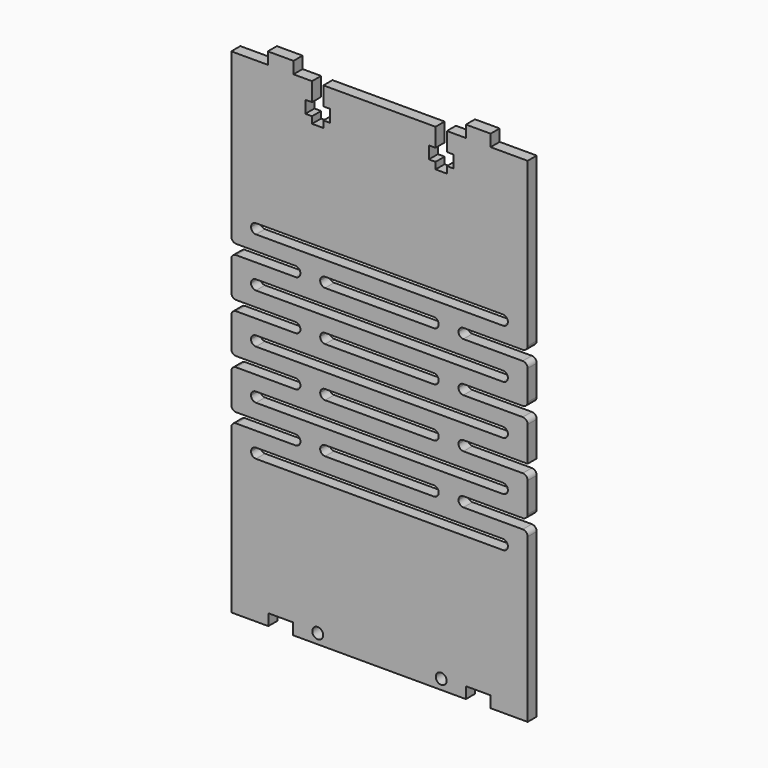
from build123d import *

# Parameters (mm, degrees)
F0_R     = 1.397
F1_DEPTH = 2.921
F2_R     = 1.26999


# Not quite as in the source:
# - a fillet or chamfer is up to 0.001 mm smaller than in the source, because OpenCascade refuses the exact size


with BuildPart() as f1:
    # F0 (on Front) → F1 (new body)
    with BuildSketch(Plane.XZ):
        Polygon((38.1, 68.58), (38.1, 64.77), (71.12, 64.77), (71.12, 63.5), (76.2, 63.5), (76.2, 68.58), (58.42, 68.58), (58.42, 71.12), (76.2, 71.12), (76.2, 81.28), (58.42, 81.28), (58.42, 83.82), (76.2, 83.82), (76.2, 127), (66.675, 127), (66.675, 123.952), (60.325, 123.952), (60.325, 127), (55.4355, 127), (55.4355, 122.2375), (57.15, 122.2375), (57.15, 119.0625), (55.4355, 119.0625), (55.4355, 117.348), (53.975, 117.348), (52.5145, 117.348), (52.5145, 119.0625), (50.8, 119.0625), (50.8, 122.2375), (52.5145, 122.2375), (52.5145, 127), (38.1, 127), (38.1, 90.17), (71.12, 90.17), (71.12, 87.63), (38.1, 87.63), (38.1, 83.82), (53.34, 83.82), (53.34, 81.28), (38.1, 81.28), (38.1, 77.47), (71.12, 77.47), (71.12, 74.93), (38.1, 74.93), (38.1, 71.12), (53.34, 71.12), (53.34, 68.58), align=None)
        Polygon((0, 68.58), (0, 63.5), (5.08, 63.5), (5.08, 64.77), (38.1, 64.77), (38.1, 68.58), (22.86, 68.58), (22.86, 71.12), (38.1, 71.12), (38.1, 74.93), (5.08, 74.93), (5.08, 77.47), (38.1, 77.47), (38.1, 81.28), (22.86, 81.28), (22.86, 83.82), (38.1, 83.82), (38.1, 87.63), (5.08, 87.63), (5.08, 90.17), (38.1, 90.17), (38.1, 127), (23.6855, 127), (23.6855, 122.2375), (25.4, 122.2375), (25.4, 119.0625), (23.6855, 119.0625), (23.6855, 117.348), (22.225, 117.348), (20.7645, 117.348), (20.7645, 119.0625), (19.05, 119.0625), (19.05, 122.2375), (20.7645, 122.2375), (20.7645, 127), (16.002, 127), (16.002, 123.952), (9.398, 123.952), (9.398, 127), (0, 127), (0, 83.82), (17.78, 83.82), (17.78, 81.28), (0, 81.28), (0, 71.12), (17.78, 71.12), (17.78, 68.58), align=None)
        Polygon((38.1, 36.83), (38.1, 0), (60.325, 0), (60.325, 2.921), (66.675, 2.921), (66.675, 0), (76.2, 0), (76.2, 43.18), (58.42, 43.18), (58.42, 45.72), (76.2, 45.72), (76.2, 55.88), (58.42, 55.88), (58.42, 58.42), (76.2, 58.42), (76.2, 63.5), (71.12, 63.5), (71.12, 62.23), (38.1, 62.23), (38.1, 58.42), (53.34, 58.42), (53.34, 55.88), (38.1, 55.88), (38.1, 52.07), (71.12, 52.07), (71.12, 49.53), (38.1, 49.53), (38.1, 45.72), (53.34, 45.72), (53.34, 43.18), (38.1, 43.18), (38.1, 39.37), (71.12, 39.37), (71.12, 36.83), align=None)
        with Locations((53.975, 2.54)):
            Circle(F0_R, mode=Mode.SUBTRACT)
        Polygon((0, 43.18), (0, 0), (9.525, 0), (9.525, 2.921), (15.875, 2.921), (15.875, 0), (38.1, 0), (38.1, 36.83), (5.08, 36.83), (5.08, 39.37), (38.1, 39.37), (38.1, 43.18), (22.86, 43.18), (22.86, 45.72), (38.1, 45.72), (38.1, 49.53), (5.08, 49.53), (5.08, 52.07), (38.1, 52.07), (38.1, 55.88), (22.86, 55.88), (22.86, 58.42), (38.1, 58.42), (38.1, 62.23), (5.08, 62.23), (5.08, 63.5), (0, 63.5), (0, 58.42), (17.78, 58.42), (17.78, 55.88), (0, 55.88), (0, 45.72), (17.78, 45.72), (17.78, 43.18), align=None)
        with Locations((22.225, 2.54)):
            Circle(F0_R, mode=Mode.SUBTRACT)
        Polygon((66.675, 123.952), (66.675, 127), (63.5, 127), (60.325, 127), (60.325, 123.952), align=None)
        Polygon((63.5, 127), (66.675, 127), (66.675, 130.048), (60.325, 130.048), (60.325, 127), align=None)
        Polygon((12.7, 127), (9.398, 127), (9.398, 123.952), (16.002, 123.952), (16.002, 127), align=None)
        Polygon((9.398, 130.048), (9.398, 127), (12.7, 127), (16.002, 127), (16.002, 130.048), align=None)
    extrude(amount=F1_DEPTH)

    # F2 (radius 1.27 in the source; OpenCascade refuses exactly that, so slightly less here)
    f2_edges = [f1.edges().sort_by_distance(p)[0] for p in [
        (76.2, -1.4605, 43.18),
        (76.2, -1.4605, 45.72),
        (76.2, -1.4605, 55.88),
        (76.2, -1.4605, 68.58),
        (76.2, -1.4605, 71.12),
        (76.2, -1.4605, 81.28),
        (76.2, -1.4605, 83.82),
        (58.42, -1.4605, 81.28),
        (58.42, -1.4605, 68.58),
        (58.42, -1.4605, 55.88),
        (58.42, -1.4605, 43.18),
        (22.86, -1.4605, 43.18),
        (22.86, -1.4605, 81.28),
        (22.86, -1.4605, 68.58),
        (22.86, -1.4605, 55.88),
        (5.08, -1.4605, 36.83),
        (5.08, -1.4605, 49.53),
        (5.08, -1.4605, 62.23),
        (5.08, -1.4605, 74.93),
        (5.08, -1.4605, 87.63),
        (71.12, -1.4605, 87.63),
        (71.12, -1.4605, 74.93),
        (71.12, -1.4605, 62.23),
        (71.12, -1.4605, 49.53),
        (71.12, -1.4605, 36.83),
        (0, -1.4605, 43.18),
        (0, -1.4605, 45.72),
        (0, -1.4605, 55.88),
        (0, -1.4605, 58.42),
        (0, -1.4605, 68.58),
        (0, -1.4605, 71.12),
        (0, -1.4605, 81.28),
        (0, -1.4605, 83.82),
        (53.34, -1.4605, 43.18),
        (53.34, -1.4605, 55.88),
        (53.34, -1.4605, 68.58),
        (53.34, -1.4605, 81.28),
        (71.12, -1.4605, 39.37),
        (71.12, -1.4605, 64.77),
        (71.12, -1.4605, 52.07),
        (71.12, -1.4605, 77.47),
        (71.12, -1.4605, 90.17),
        (53.34, -1.4605, 83.82),
        (53.34, -1.4605, 58.42),
        (53.34, -1.4605, 45.72),
        (17.78, -1.4605, 45.72),
        (17.78, -1.4605, 58.42),
        (17.78, -1.4605, 71.12),
        (17.78, -1.4605, 83.82),
        (5.08, -1.4605, 39.37),
        (5.08, -1.4605, 52.07),
        (5.08, -1.4605, 64.77),
        (5.08, -1.4605, 77.47),
        (5.08, -1.4605, 90.17),
        (22.86, -1.4605, 45.72),
        (22.86, -1.4605, 58.42),
        (22.86, -1.4605, 83.82),
        (22.86, -1.4605, 71.12),
        (53.34, -1.4605, 71.12),
        (17.78, -1.4605, 43.18),
        (17.78, -1.4605, 55.88),
        (17.78, -1.4605, 68.58),
        (17.78, -1.4605, 81.28),
        (58.42, -1.4605, 45.72),
        (58.42, -1.4605, 58.42),
        (58.42, -1.4605, 71.12),
        (58.42, -1.4605, 83.82),
    ]]
    fillet(f2_edges, radius=F2_R)


solid = f1.part
